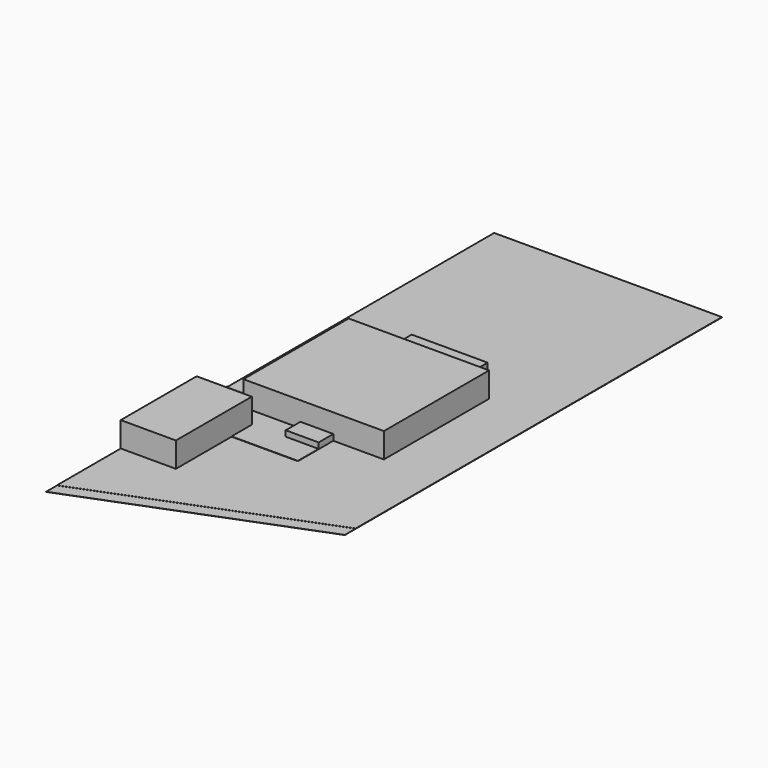
from build123d import *

# Parameters (mm, degrees)
F3_DEPTH  = 25
F1_W      = 11100
F1_H      = 10390
F4_DEPTH  = 25
F5_DEPTH  = 10
F0_W      = 11100
F0_H      = 10390
F0_W_2    = 4360
F0_H_2    = 7500
F6_DEPTH  = 2000
F2_W      = 2600
F2_H      = 1450
F2_W_2    = 6000
F2_H_2    = 3000
F7_DEPTH  = 500
F8_DEPTH  = 50
F9_W      = 2500
F9_H      = 1500
F10_DEPTH = 25
F11_W     = 1300
F11_H     = 4800
F12_DEPTH = 1000


with BuildPart() as f3:
    # F2 (on face) → F3 (new body)
    with BuildSketch(Plane.XY):
        Polygon((5660, -36890), (4360, -36890), (0, -36890), (0, -43190), (5660, -40984.2647058823), align=None)
    extrude(amount=F3_DEPTH)


with BuildPart() as f4:
    # F1 (on face) → F4 (new body)
    with BuildSketch(Plane.XY):
        Polygon((18000, 0), (0, 0), (0, -29390), (4360, -29390), (4360, -36890), (0, -36890), (0, -43190), (18000, -36175.2941176471), align=None)
        with Locations((8050, -22695)):
            Rectangle(F1_W, F1_H, mode=Mode.SUBTRACT)
    extrude(amount=F4_DEPTH)

    # F0 (on Top) → F5 (join)
    with BuildSketch(Plane.XY):
        Polygon((18000, -37248.5464993078), (18000, -36175.2941176471), (0, -43190), (0, -44263.2523816607), align=None)
    extrude(amount=F5_DEPTH)

    # F0 (on Top) → F6 (join)
    with BuildSketch(Plane.XY):
        with Locations((8050, -22695)):
            Rectangle(F0_W, F0_H)
        with Locations((2180, -33140)):
            Rectangle(F0_W_2, F0_H_2)
    extrude(amount=F6_DEPTH)

    # F2 (on face) → F7 (join)
    with BuildSketch(Plane.XY):
        with Locations((8300, -28615)):
            Rectangle(F2_W, F2_H)
        with Locations((8086.6937637329, -16000)):
            Rectangle(F2_W_2, F2_H_2)
    extrude(amount=F7_DEPTH)

    # F2 (on face) → F8 (join)
    with BuildSketch(Plane.XY):
        Polygon((7000, -29340), (7000, -27890), (2500, -27890), (2500, -26390), (0, -26390), (0, -29390), (4360, -29390), (4360, -31390), (9600, -31390), (9600, -29340), align=None)
    extrude(amount=F8_DEPTH)

    # F9 (on face) → F10 (join)
    with BuildSketch(Plane.XY.offset(50)):
        with Locations((1250, -27140)):
            Rectangle(F9_W, F9_H)
    extrude(amount=F10_DEPTH)

    # F11 (on Top) → F12 (join)
    with BuildSketch(Plane.XY):
        with Locations((1850, -21300)):
            Rectangle(F11_W, F11_H)
    extrude(amount=F12_DEPTH)


solid = Compound([f3.part, f4.part])
